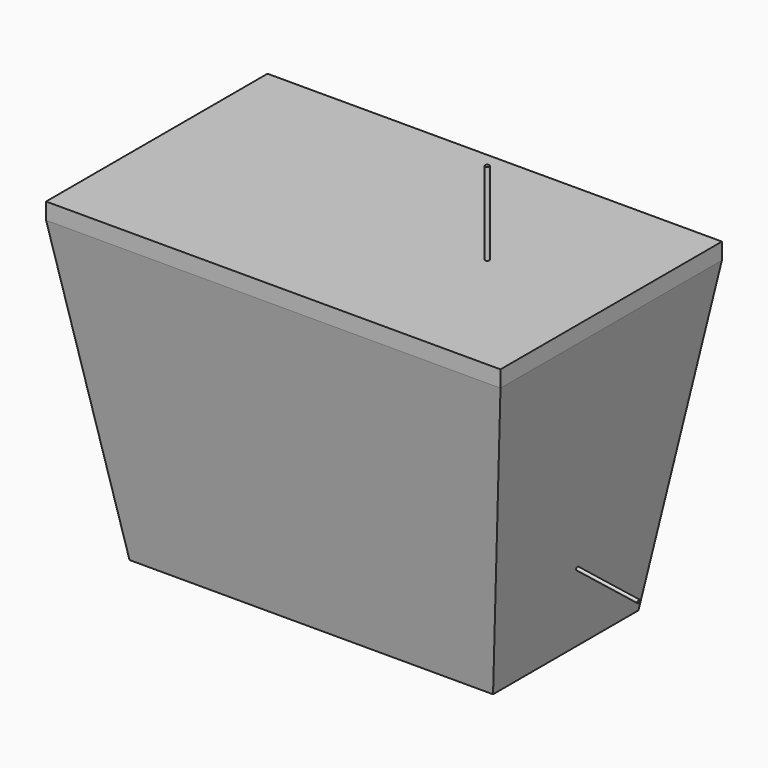
from build123d import *

# Parameters (mm, degrees)
F2_W      = 440
F2_H      = 220
F3_W      = 550
F3_H      = 335
F5_T      = -15
F6_R      = 10
F7_DEPTH  = 160
F8_W      = 10
F8_H      = 0.5
F8_W_2    = 310.5556852937
F8_W_3    = 330.5556852937
F8_H_2    = 7.628889712
F8_W_4    = 350.5556852937
F7_FACE_R = 10
F9_DEPTH  = 1
F8_H_3    = 8
F10_DEPTH = 19.05
F11_W     = 0.5
F11_H     = 137.0105478786
F12_DEPTH = 1
F13_R     = 50
F14_DEPTH = 150
F15_R     = 37.5
F16_DEPTH = 30
F17_R     = 5
F18_R     = 40
F19_DEPTH = 20
F20_R     = 18.75
F21_DEPTH = 25
F25_W     = 550
F25_H     = 335
F26_DEPTH = 20
F27_R     = 1.987683668
F28_DEPTH = 75
F29_R     = 2.5
F30_DEPTH = 100


with BuildPart() as f4:
    # F2 (on offset) → F4 section 0
    with BuildSketch(Plane.XY.offset(-167.5)):
        Rectangle(F2_W, F2_H)
    # F3 (on offset) → F4 section 1
    with BuildSketch(Plane.XY.offset(200)):
        Rectangle(F3_W, F3_H)
    loft()

    # F5
    f5_openings = [f4.faces().sort_by_distance(p)[0] for p in [
        (0, 0, 200),
    ]]
    offset(amount=F5_T, openings=f5_openings)

    # F6 (on face) → F7 (join)
    with BuildSketch(Plane.XY.offset(-152.5)):
        with Locations((-155.2778426469, 48.564444856)):
            Circle(F6_R)
        with Locations((-155.2778426469, -48.564444856)):
            Circle(F6_R)
        with Locations((155.2778426469, 48.564444856)):
            Circle(F6_R)
        with Locations((155.2778426469, -48.564444856)):
            Circle(F6_R)
    extrude(amount=F7_DEPTH)

    # F8 (on face) + F7_face (on face) + F6 (on face) → F9 (join)
    with BuildSketch(Plane.XY.offset(7.5)):
        Polygon((-165.2778426469, -58.564444856), (-165.2778426469, -50.935555144), (-175.2778426469, -50.935555144), (-175.2778426469, -58.935555144), (175.2778426469, -58.935555144), (175.2778426469, -50.935555144), (165.2778426469, -50.935555144), (165.2778426469, -58.564444856), align=None)
        with Locations((-170.2778426469, 0.314444856)):
            Rectangle(F8_W, F8_H)
        with Locations((-170.2778426469, 25.814444856)):
            Rectangle(F8_W, F8_H)
        with Locations((160.2778426469, 25.814444856)):
            Rectangle(F8_W, F8_H)
        with Locations((-160.2778426469, 25.814444856)):
            Rectangle(F8_W, F8_H)
        with Locations((-160.2778426469, -33.685555144)):
            Rectangle(F8_W, F8_H)
        with Locations((-160.2778426469, 0.314444856)):
            Rectangle(F8_W, F8_H)
        with Locations((0, 8.814444856)):
            Rectangle(F8_W_2, F8_H)
        with Locations((0, -25.185555144)):
            Rectangle(F8_W_2, F8_H)
        with Locations((-160.2778426469, 34.314444856)):
            Rectangle(F8_W, F8_H)
        with BuildLine():
            ThreePointArc((-145.7384506327, 51.564444856), (-145.6636664989, 51.3153750614), (-145.5953842813, 51.064444856))
            Line((-145.5953842813, 51.064444856), (165.2778426469, 51.064444856))
            Line((165.2778426469, 51.064444856), (165.2778426469, 51.564444856))
            Line((165.2778426469, 51.564444856), (-145.7384506327, 51.564444856))
        make_face()
        with Locations((160.2778426469, 0.314444856)):
            Rectangle(F8_W, F8_H)
        with Locations((-160.2778426469, -16.685555144)):
            Rectangle(F8_W, F8_H)
        with Locations((160.2778426469, -8.185555144)):
            Rectangle(F8_W, F8_H)
        with Locations((-170.2778426469, -42.185555144)):
            Rectangle(F8_W, F8_H)
        with Locations((160.2778426469, -25.185555144)):
            Rectangle(F8_W, F8_H)
        with Locations((-160.2778426469, -8.185555144)):
            Rectangle(F8_W, F8_H)
        with Locations((0, -42.185555144)):
            Rectangle(F8_W_2, F8_H)
        with Locations((-170.2778426469, 8.814444856)):
            Rectangle(F8_W, F8_H)
        with Locations((0, 0.314444856)):
            Rectangle(F8_W_2, F8_H)
        with Locations((160.2778426469, -16.685555144)):
            Rectangle(F8_W, F8_H)
        with Locations((160.2778426469, 8.814444856)):
            Rectangle(F8_W, F8_H)
        with Locations((0, -33.685555144)):
            Rectangle(F8_W_2, F8_H)
        with Locations((-170.2778426469, -8.185555144)):
            Rectangle(F8_W, F8_H)
        with Locations((-160.2778426469, 17.314444856)):
            Rectangle(F8_W, F8_H)
        with Locations((0, 34.314444856)):
            Rectangle(F8_W_2, F8_H)
        with Locations((-170.2778426469, -16.685555144)):
            Rectangle(F8_W, F8_H)
        with Locations((160.2778426469, -33.685555144)):
            Rectangle(F8_W, F8_H)
        with Locations((160.2778426469, 34.314444856)):
            Rectangle(F8_W, F8_H)
        with BuildLine():
            Line((-145.2778426469, 48.564444856), (-155.2778426469, 48.564444856))
            Line((-155.2778426469, 48.564444856), (-155.2778426469, 43.064444856))
            Line((-155.2778426469, 43.064444856), (-146.9261961026, 43.064444856))
            ThreePointArc((-146.9261961026, 43.064444856), (-145.6987908816, 45.6935970233), (-145.2778426469, 48.564444856))
        make_face()
        with Locations((0, -54.75)):
            Rectangle(F8_W_3, F8_H_2)
        with BuildLine():
            Line((155.2778426469, 43.064444856), (-146.9261961026, 43.064444856))
            ThreePointArc((-146.9261961026, 43.064444856), (-147.0981980227, 42.8117573255), (-147.2778426469, 42.564444856))
            Line((-147.2778426469, 42.564444856), (155.2778426469, 42.564444856))
            Line((155.2778426469, 42.564444856), (155.2778426469, 43.064444856))
        make_face()
        with BuildLine():
            Line((-164.817234661, 51.564444856), (-145.7384506327, 51.564444856))
            ThreePointArc((-145.7384506327, 51.564444856), (-149.3617628638, 56.6267026043), (-155.2778426469, 58.564444856))
            ThreePointArc((-155.2778426469, 58.564444856), (-161.19392243, 56.6267026043), (-164.817234661, 51.564444856))
        make_face()
        with Locations((0, 25.814444856)):
            Rectangle(F8_W_2, F8_H)
        with Locations((0, -8.185555144)):
            Rectangle(F8_W_2, F8_H)
        with Locations((160.2778426469, 42.814444856)):
            Rectangle(F8_W, F8_H)
        with Locations((160.2778426469, 17.314444856)):
            Rectangle(F8_W, F8_H)
        with Locations((-170.2778426469, -50.685555144)):
            Rectangle(F8_W, F8_H)
        with Locations((-170.2778426469, 17.314444856)):
            Rectangle(F8_W, F8_H)
        with Locations((-170.2778426469, 51.314444856)):
            Rectangle(F8_W, F8_H)
        with Locations((-160.2778426469, -25.185555144)):
            Rectangle(F8_W, F8_H)
        with Locations((-160.2778426469, 8.814444856)):
            Rectangle(F8_W, F8_H)
        with Locations((160.2778426469, -42.185555144)):
            Rectangle(F8_W, F8_H)
        with Locations((-170.2778426469, 34.314444856)):
            Rectangle(F8_W, F8_H)
        with Locations((-170.2778426469, -33.685555144)):
            Rectangle(F8_W, F8_H)
        with BuildLine():
            Line((-155.2778426469, 42.564444856), (-155.2778426469, 43.064444856))
            Line((-155.2778426469, 43.064444856), (-163.6294891911, 43.064444856))
            ThreePointArc((-163.6294891911, 43.064444856), (-163.457487271, 42.8117573255), (-163.2778426469, 42.564444856))
            Line((-163.2778426469, 42.564444856), (-155.2778426469, 42.564444856))
        make_face()
        with Locations((-170.2778426469, -25.185555144)):
            Rectangle(F8_W, F8_H)
        with Locations((-170.2778426469, 42.814444856)):
            Rectangle(F8_W, F8_H)
        with Locations((0, -16.685555144)):
            Rectangle(F8_W_2, F8_H)
        with Locations((0, 17.314444856)):
            Rectangle(F8_W_2, F8_H)
        with BuildLine():
            Line((-147.2778426469, 42.564444856), (-155.2778426469, 42.564444856))
            Line((-155.2778426469, 42.564444856), (-155.2778426469, 38.564444856))
            ThreePointArc((-155.2778426469, 38.564444856), (-150.8057066919, 39.620172946), (-147.2778426469, 42.564444856))
        make_face()
        with Locations((-160.2778426469, -42.185555144)):
            Rectangle(F8_W, F8_H)
        with BuildLine():
            Line((-155.2778426469, 43.064444856), (-155.2778426469, 48.564444856))
            Line((-155.2778426469, 48.564444856), (-145.2778426469, 48.564444856))
            ThreePointArc((-145.2778426469, 48.564444856), (-145.3575456842, 49.8244877808), (-145.5953842813, 51.064444856))
            Line((-145.5953842813, 51.064444856), (-164.9603010124, 51.064444856))
            ThreePointArc((-164.9603010124, 51.064444856), (-165.1981396095, 49.8244877808), (-165.2778426469, 48.564444856))
            ThreePointArc((-165.2778426469, 48.564444856), (-164.8568944121, 45.6935970233), (-163.6294891911, 43.064444856))
            Line((-163.6294891911, 43.064444856), (-155.2778426469, 43.064444856))
        make_face()
        with BuildLine():
            Line((-146.9261961026, 43.064444856), (-155.2778426469, 43.064444856))
            Line((-155.2778426469, 43.064444856), (-155.2778426469, 42.564444856))
            Line((-155.2778426469, 42.564444856), (-147.2778426469, 42.564444856))
            ThreePointArc((-147.2778426469, 42.564444856), (-147.0981980227, 42.8117573255), (-146.9261961026, 43.064444856))
        make_face()
        with Locations((0, -50.685555144)):
            Rectangle(F8_W_3, F8_H)
        with BuildLine():
            Line((-155.2778426469, 38.564444856), (-155.2778426469, 42.564444856))
            Line((-155.2778426469, 42.564444856), (-163.2778426469, 42.564444856))
            ThreePointArc((-163.2778426469, 42.564444856), (-159.7499786019, 39.620172946), (-155.2778426469, 38.564444856))
        make_face()
        with BuildLine():
            Line((-164.9603010124, 51.064444856), (-145.5953842813, 51.064444856))
            ThreePointArc((-145.5953842813, 51.064444856), (-145.6636664989, 51.3153750614), (-145.7384506327, 51.564444856))
            Line((-145.7384506327, 51.564444856), (-164.817234661, 51.564444856))
            ThreePointArc((-164.817234661, 51.564444856), (-164.8920187949, 51.3153750614), (-164.9603010124, 51.064444856))
        make_face()
        with BuildLine():
            ThreePointArc((-163.2778426469, 42.564444856), (-163.457487271, 42.8117573255), (-163.6294891911, 43.064444856))
            Line((-163.6294891911, 43.064444856), (-165.2778426469, 43.064444856))
            Line((-165.2778426469, 43.064444856), (-165.2778426469, 42.564444856))
            Line((-165.2778426469, 42.564444856), (-163.2778426469, 42.564444856))
        make_face()
        with BuildLine():
            Line((-165.2778426469, 51.064444856), (-164.9603010124, 51.064444856))
            ThreePointArc((-164.9603010124, 51.064444856), (-164.8920187949, 51.3153750614), (-164.817234661, 51.564444856))
            Line((-164.817234661, 51.564444856), (-165.2778426469, 51.564444856))
            Line((-165.2778426469, 51.564444856), (-165.2778426469, 51.064444856))
        make_face()
        with Locations((0, 68.314444856)):
            Rectangle(F8_W_4, F8_H)
        with Locations((0, 59.814444856)):
            Rectangle(F8_W_4, F8_H)
    with BuildSketch(Plane(origin=(-155.2778426469, 48.564444856, 7.5), x_dir=(1, 0, 0), z_dir=(0, 0, 1))):
        with Locations((310.5556852937, -97.128889712)):
            Circle(F7_FACE_R)
        with Locations((0, -97.128889712)):
            Circle(F7_FACE_R)
        Circle(F7_FACE_R)
        with Locations((310.5556852937, 0)):
            Circle(F7_FACE_R)
    with BuildSketch(Plane.XY.offset(-152.5)):
        with Locations((-155.2778426469, -48.564444856)):
            Circle(F6_R)
        with Locations((155.2778426469, -48.564444856)):
            Circle(F6_R)
        with Locations((155.2778426469, 48.564444856)):
            Circle(F6_R)
        with Locations((-155.2778426469, 48.564444856)):
            Circle(F6_R)
    extrude(amount=-F9_DEPTH)

    # F18 (on face) → F19 (join)
    with BuildSketch(Plane.XY.offset(-152.5)):
        Circle(F18_R)
    extrude(amount=F19_DEPTH)

    # F20 (on face) → F21 (join)
    with BuildSketch(Plane.XY.offset(-132.5)):
        Circle(F20_R)
    extrude(amount=F21_DEPTH)

    # F23 (on face) → F24 (revolve)
    with BuildSketch(Plane(origin=(0, 0, 0), x_dir=(0, -1, 0), z_dir=(-1, 0, 0))):
        with BuildLine():
            Line((0, -40), (0, -120))
            ThreePointArc((0, -120), (45.3792520632, -80), (0, -40))
        make_face()
    revolve(axis=Axis((0, 0, -80), (0, 0, -1)))

    # F25 (on face) → F26 (join)
    with BuildSketch(Plane.XY.offset(200)):
        Rectangle(F25_W, F25_H)
    extrude(amount=F26_DEPTH)

    # F27 (on face) → F28 (join, symmetric)
    with BuildSketch(Plane(origin=(239.6992259992, 0, -35.8733535509), x_dir=(0, 1, 0), z_dir=(0.9889856463, 0, -0.1480114573))):
        with Locations((0, -38.0925751513)):
            Circle(F27_R)
    extrude(amount=F28_DEPTH, both=True)


with BuildPart() as f10:
    # F8 (on face) → F10 (new body)
    with BuildSketch(Plane.XY.offset(7.5)):
        with Locations((0, -64.564444856)):
            Rectangle(F8_W_4, F8_H_3)
    extrude(amount=-F10_DEPTH)


with BuildPart() as f10b:
    # F8 (on face) → F10, piece 2 (new body)
    with BuildSketch(Plane.XY.offset(7.5)):
        Polygon((-165.2778426469, -58.564444856), (-165.2778426469, -50.935555144), (-175.2778426469, -50.935555144), (-175.2778426469, -58.935555144), (175.2778426469, -58.935555144), (175.2778426469, -50.935555144), (165.2778426469, -50.935555144), (165.2778426469, -58.564444856), align=None)
    extrude(amount=-F10_DEPTH)


with BuildPart() as f10c:
    # F8 (on face) → F10, piece 3 (new body)
    with BuildSketch(Plane.XY.offset(7.5)):
        with Locations((170.2778426469, -46.435555144)):
            Rectangle(F8_W, F8_H_3)
    extrude(amount=-F10_DEPTH)


with BuildPart() as f10d:
    # F8 (on face) → F10, piece 4 (new body)
    with BuildSketch(Plane.XY.offset(7.5)):
        with Locations((170.2778426469, -37.935555144)):
            Rectangle(F8_W, F8_H_3)
    extrude(amount=-F10_DEPTH)


with BuildPart() as f10e:
    # F8 (on face) → F10, piece 5 (new body)
    with BuildSketch(Plane.XY.offset(7.5)):
        with Locations((170.2778426469, -29.435555144)):
            Rectangle(F8_W, F8_H_3)
    extrude(amount=-F10_DEPTH)


with BuildPart() as f10f:
    # F8 (on face) → F10, piece 6 (new body)
    with BuildSketch(Plane.XY.offset(7.5)):
        with Locations((170.2778426469, -20.935555144)):
            Rectangle(F8_W, F8_H_3)
    extrude(amount=-F10_DEPTH)


with BuildPart() as f10g:
    # F8 (on face) → F10, piece 7 (new body)
    with BuildSketch(Plane.XY.offset(7.5)):
        with Locations((170.2778426469, -12.435555144)):
            Rectangle(F8_W, F8_H_3)
    extrude(amount=-F10_DEPTH)


with BuildPart() as f10h:
    # F8 (on face) → F10, piece 8 (new body)
    with BuildSketch(Plane.XY.offset(7.5)):
        with Locations((170.2778426469, -3.935555144)):
            Rectangle(F8_W, F8_H_3)
    extrude(amount=-F10_DEPTH)


with BuildPart() as f10i:
    # F8 (on face) → F10, piece 9 (new body)
    with BuildSketch(Plane.XY.offset(7.5)):
        with Locations((170.2778426469, 4.564444856)):
            Rectangle(F8_W, F8_H_3)
    extrude(amount=-F10_DEPTH)


with BuildPart() as f10j:
    # F8 (on face) → F10, piece 10 (new body)
    with BuildSketch(Plane.XY.offset(7.5)):
        with Locations((170.2778426469, 13.064444856)):
            Rectangle(F8_W, F8_H_3)
    extrude(amount=-F10_DEPTH)


with BuildPart() as f10k:
    # F8 (on face) → F10, piece 11 (new body)
    with BuildSketch(Plane.XY.offset(7.5)):
        with Locations((170.2778426469, 21.564444856)):
            Rectangle(F8_W, F8_H_3)
    extrude(amount=-F10_DEPTH)


with BuildPart() as f10l:
    # F8 (on face) → F10, piece 12 (new body)
    with BuildSketch(Plane.XY.offset(7.5)):
        with Locations((170.2778426469, 30.064444856)):
            Rectangle(F8_W, F8_H_3)
    extrude(amount=-F10_DEPTH)


with BuildPart() as f10m:
    # F8 (on face) → F10, piece 13 (new body)
    with BuildSketch(Plane.XY.offset(7.5)):
        with Locations((170.2778426469, 38.564444856)):
            Rectangle(F8_W, F8_H_3)
    extrude(amount=-F10_DEPTH)


with BuildPart() as f10n:
    # F8 (on face) → F10, piece 14 (new body)
    with BuildSketch(Plane.XY.offset(7.5)):
        with Locations((170.2778426469, 47.064444856)):
            Rectangle(F8_W, F8_H_3)
    extrude(amount=-F10_DEPTH)


with BuildPart() as f10o:
    # F8 (on face) → F10, piece 15 (new body)
    with BuildSketch(Plane.XY.offset(7.5)):
        Polygon((165.2778426469, 58.564444856), (165.2778426469, 51.564444856), (175.2778426469, 51.564444856), (175.2778426469, 59.564444856), (-175.2778426469, 59.564444856), (-175.2778426469, 51.564444856), (-165.2778426469, 51.564444856), (-165.2778426469, 58.564444856), (-155.2778426469, 58.564444856), align=None)
    extrude(amount=-F10_DEPTH)


with BuildPart() as f10p:
    # F8 (on face) → F10, piece 16 (new body)
    with BuildSketch(Plane.XY.offset(7.5)):
        with Locations((0, 64.064444856)):
            Rectangle(F8_W_4, F8_H_3)
    extrude(amount=-F10_DEPTH)


with BuildPart() as f10q:
    # F8 (on face) → F10, piece 17 (new body)
    with BuildSketch(Plane.XY.offset(7.5)):
        Polygon((-175.2778426469, 43.064444856), (-165.2778426469, 43.064444856), (-165.2778426469, 48.564444856), (-165.2778426469, 51.064444856), (-175.2778426469, 51.064444856), align=None)
    extrude(amount=-F10_DEPTH)


with BuildPart() as f10r:
    # F8 (on face) → F10, piece 18 (new body)
    with BuildSketch(Plane.XY.offset(7.5)):
        with Locations((-170.2778426469, 38.564444856)):
            Rectangle(F8_W, F8_H_3)
    extrude(amount=-F10_DEPTH)


with BuildPart() as f10s:
    # F8 (on face) → F10, piece 19 (new body)
    with BuildSketch(Plane.XY.offset(7.5)):
        with Locations((-170.2778426469, 30.064444856)):
            Rectangle(F8_W, F8_H_3)
    extrude(amount=-F10_DEPTH)


with BuildPart() as f10t:
    # F8 (on face) → F10, piece 20 (new body)
    with BuildSketch(Plane.XY.offset(7.5)):
        with Locations((-170.2778426469, 21.564444856)):
            Rectangle(F8_W, F8_H_3)
    extrude(amount=-F10_DEPTH)


with BuildPart() as f10u:
    # F8 (on face) → F10, piece 21 (new body)
    with BuildSketch(Plane.XY.offset(7.5)):
        with Locations((-170.2778426469, 13.064444856)):
            Rectangle(F8_W, F8_H_3)
    extrude(amount=-F10_DEPTH)


with BuildPart() as f10v:
    # F8 (on face) → F10, piece 22 (new body)
    with BuildSketch(Plane.XY.offset(7.5)):
        with Locations((-170.2778426469, 4.564444856)):
            Rectangle(F8_W, F8_H_3)
    extrude(amount=-F10_DEPTH)


with BuildPart() as f10w:
    # F8 (on face) → F10, piece 23 (new body)
    with BuildSketch(Plane.XY.offset(7.5)):
        with Locations((-170.2778426469, -3.935555144)):
            Rectangle(F8_W, F8_H_3)
    extrude(amount=-F10_DEPTH)


with BuildPart() as f10x:
    # F8 (on face) → F10, piece 24 (new body)
    with BuildSketch(Plane.XY.offset(7.5)):
        with Locations((-170.2778426469, -12.435555144)):
            Rectangle(F8_W, F8_H_3)
    extrude(amount=-F10_DEPTH)


with BuildPart() as f10y:
    # F8 (on face) → F10, piece 25 (new body)
    with BuildSketch(Plane.XY.offset(7.5)):
        with Locations((-170.2778426469, -20.935555144)):
            Rectangle(F8_W, F8_H_3)
    extrude(amount=-F10_DEPTH)


with BuildPart() as f10z:
    # F8 (on face) → F10, piece 26 (new body)
    with BuildSketch(Plane.XY.offset(7.5)):
        with Locations((-170.2778426469, -29.435555144)):
            Rectangle(F8_W, F8_H_3)
    extrude(amount=-F10_DEPTH)


with BuildPart() as f10ba:
    # F8 (on face) → F10, piece 27 (new body)
    with BuildSketch(Plane.XY.offset(7.5)):
        with Locations((-170.2778426469, -37.935555144)):
            Rectangle(F8_W, F8_H_3)
    extrude(amount=-F10_DEPTH)


with BuildPart() as f10bb:
    # F8 (on face) → F10, piece 28 (new body)
    with BuildSketch(Plane.XY.offset(7.5)):
        with Locations((-170.2778426469, -46.435555144)):
            Rectangle(F8_W, F8_H_3)
    extrude(amount=-F10_DEPTH)


with BuildPart() as f12:
    # F11 (on face) → F12 (new body)
    with BuildSketch(Plane.XY.offset(7.5)):
        with Locations((-175.0278426469, -0.4408290833)):
            Rectangle(F11_W, F11_H)
    extrude(amount=-F12_DEPTH)


with BuildPart() as f12b:
    # F11 (on face) → F12, piece 2 (new body)
    with BuildSketch(Plane.XY.offset(7.5)):
        with Locations((-167.0278426469, -0.4408290833)):
            Rectangle(F11_W, F11_H)
    extrude(amount=-F12_DEPTH)


with BuildPart() as f12c:
    # F11 (on face) → F12, piece 3 (new body)
    with BuildSketch(Plane.XY.offset(7.5)):
        with Locations((-159.0278426469, -0.4408290833)):
            Rectangle(F11_W, F11_H)
    extrude(amount=-F12_DEPTH)


with BuildPart() as f12d:
    # F11 (on face) → F12, piece 4 (new body)
    with BuildSketch(Plane.XY.offset(7.5)):
        with Locations((-151.0278426469, -0.4408290833)):
            Rectangle(F11_W, F11_H)
    extrude(amount=-F12_DEPTH)


with BuildPart() as f12e:
    # F11 (on face) → F12, piece 5 (new body)
    with BuildSketch(Plane.XY.offset(7.5)):
        with Locations((-143.0278426469, -0.4408290833)):
            Rectangle(F11_W, F11_H)
    extrude(amount=-F12_DEPTH)


with BuildPart() as f12f:
    # F11 (on face) → F12, piece 6 (new body)
    with BuildSketch(Plane.XY.offset(7.5)):
        with Locations((-135.0278426469, -0.4408290833)):
            Rectangle(F11_W, F11_H)
    extrude(amount=-F12_DEPTH)


with BuildPart() as f12g:
    # F11 (on face) → F12, piece 7 (new body)
    with BuildSketch(Plane.XY.offset(7.5)):
        with Locations((-127.0278426469, -0.4408290833)):
            Rectangle(F11_W, F11_H)
    extrude(amount=-F12_DEPTH)


with BuildPart() as f12h:
    # F11 (on face) → F12, piece 8 (new body)
    with BuildSketch(Plane.XY.offset(7.5)):
        with Locations((-119.0278426469, -0.4408290833)):
            Rectangle(F11_W, F11_H)
    extrude(amount=-F12_DEPTH)


with BuildPart() as f12i:
    # F11 (on face) → F12, piece 9 (new body)
    with BuildSketch(Plane.XY.offset(7.5)):
        with Locations((-111.0278426469, -0.4408290833)):
            Rectangle(F11_W, F11_H)
    extrude(amount=-F12_DEPTH)


with BuildPart() as f12j:
    # F11 (on face) → F12, piece 10 (new body)
    with BuildSketch(Plane.XY.offset(7.5)):
        with Locations((-103.0278426469, -0.4408290833)):
            Rectangle(F11_W, F11_H)
    extrude(amount=-F12_DEPTH)


with BuildPart() as f12k:
    # F11 (on face) → F12, piece 11 (new body)
    with BuildSketch(Plane.XY.offset(7.5)):
        with Locations((-95.0278426469, -0.4408290833)):
            Rectangle(F11_W, F11_H)
    extrude(amount=-F12_DEPTH)


with BuildPart() as f12l:
    # F11 (on face) → F12, piece 12 (new body)
    with BuildSketch(Plane.XY.offset(7.5)):
        with Locations((-87.0278426469, -0.4408290833)):
            Rectangle(F11_W, F11_H)
    extrude(amount=-F12_DEPTH)


with BuildPart() as f12m:
    # F11 (on face) → F12, piece 13 (new body)
    with BuildSketch(Plane.XY.offset(7.5)):
        with Locations((-79.0278426469, -0.4408290833)):
            Rectangle(F11_W, F11_H)
    extrude(amount=-F12_DEPTH)


with BuildPart() as f12n:
    # F11 (on face) → F12, piece 14 (new body)
    with BuildSketch(Plane.XY.offset(7.5)):
        with Locations((-71.0278426469, -0.4408290833)):
            Rectangle(F11_W, F11_H)
    extrude(amount=-F12_DEPTH)


with BuildPart() as f12o:
    # F11 (on face) → F12, piece 15 (new body)
    with BuildSketch(Plane.XY.offset(7.5)):
        with Locations((-63.0278426469, -0.4408290833)):
            Rectangle(F11_W, F11_H)
    extrude(amount=-F12_DEPTH)


with BuildPart() as f12p:
    # F11 (on face) → F12, piece 16 (new body)
    with BuildSketch(Plane.XY.offset(7.5)):
        with Locations((-55.0278426469, -0.4408290833)):
            Rectangle(F11_W, F11_H)
    extrude(amount=-F12_DEPTH)


with BuildPart() as f12q:
    # F11 (on face) → F12, piece 17 (new body)
    with BuildSketch(Plane.XY.offset(7.5)):
        with Locations((-47.0278426469, -0.4408290833)):
            Rectangle(F11_W, F11_H)
    extrude(amount=-F12_DEPTH)


with BuildPart() as f12r:
    # F11 (on face) → F12, piece 18 (new body)
    with BuildSketch(Plane.XY.offset(7.5)):
        with Locations((-39.0278426469, -0.4408290833)):
            Rectangle(F11_W, F11_H)
    extrude(amount=-F12_DEPTH)


with BuildPart() as f12s:
    # F11 (on face) → F12, piece 19 (new body)
    with BuildSketch(Plane.XY.offset(7.5)):
        with Locations((-31.0278426469, -0.4408290833)):
            Rectangle(F11_W, F11_H)
    extrude(amount=-F12_DEPTH)


with BuildPart() as f12t:
    # F11 (on face) → F12, piece 20 (new body)
    with BuildSketch(Plane.XY.offset(7.5)):
        with Locations((-23.0278426469, -0.4408290833)):
            Rectangle(F11_W, F11_H)
    extrude(amount=-F12_DEPTH)


with BuildPart() as f12u:
    # F11 (on face) → F12, piece 21 (new body)
    with BuildSketch(Plane.XY.offset(7.5)):
        with Locations((-15.0278426469, -0.4408290833)):
            Rectangle(F11_W, F11_H)
    extrude(amount=-F12_DEPTH)


with BuildPart() as f12v:
    # F11 (on face) → F12, piece 22 (new body)
    with BuildSketch(Plane.XY.offset(7.5)):
        with Locations((-7.0278426469, -0.4408290833)):
            Rectangle(F11_W, F11_H)
    extrude(amount=-F12_DEPTH)


with BuildPart() as f12w:
    # F11 (on face) → F12, piece 23 (new body)
    with BuildSketch(Plane.XY.offset(7.5)):
        with Locations((0.9721573531, -0.4408290833)):
            Rectangle(F11_W, F11_H)
    extrude(amount=-F12_DEPTH)


with BuildPart() as f12x:
    # F11 (on face) → F12, piece 24 (new body)
    with BuildSketch(Plane.XY.offset(7.5)):
        with Locations((8.9721573531, -0.4408290833)):
            Rectangle(F11_W, F11_H)
    extrude(amount=-F12_DEPTH)


with BuildPart() as f12y:
    # F11 (on face) → F12, piece 25 (new body)
    with BuildSketch(Plane.XY.offset(7.5)):
        with Locations((16.9721573531, -0.4408290833)):
            Rectangle(F11_W, F11_H)
    extrude(amount=-F12_DEPTH)


with BuildPart() as f12z:
    # F11 (on face) → F12, piece 26 (new body)
    with BuildSketch(Plane.XY.offset(7.5)):
        with Locations((24.9721573531, -0.4408290833)):
            Rectangle(F11_W, F11_H)
    extrude(amount=-F12_DEPTH)


with BuildPart() as f12ba:
    # F11 (on face) → F12, piece 27 (new body)
    with BuildSketch(Plane.XY.offset(7.5)):
        with Locations((32.9721573531, -0.4408290833)):
            Rectangle(F11_W, F11_H)
    extrude(amount=-F12_DEPTH)


with BuildPart() as f12bb:
    # F11 (on face) → F12, piece 28 (new body)
    with BuildSketch(Plane.XY.offset(7.5)):
        with Locations((40.9721573531, -0.4408290833)):
            Rectangle(F11_W, F11_H)
    extrude(amount=-F12_DEPTH)


with BuildPart() as f12bc:
    # F11 (on face) → F12, piece 29 (new body)
    with BuildSketch(Plane.XY.offset(7.5)):
        with Locations((48.9721573531, -0.4408290833)):
            Rectangle(F11_W, F11_H)
    extrude(amount=-F12_DEPTH)


with BuildPart() as f12bd:
    # F11 (on face) → F12, piece 30 (new body)
    with BuildSketch(Plane.XY.offset(7.5)):
        with Locations((56.9721573531, -0.4408290833)):
            Rectangle(F11_W, F11_H)
    extrude(amount=-F12_DEPTH)


with BuildPart() as f12be:
    # F11 (on face) → F12, piece 31 (new body)
    with BuildSketch(Plane.XY.offset(7.5)):
        with Locations((64.9721573531, -0.4408290833)):
            Rectangle(F11_W, F11_H)
    extrude(amount=-F12_DEPTH)


with BuildPart() as f12bf:
    # F11 (on face) → F12, piece 32 (new body)
    with BuildSketch(Plane.XY.offset(7.5)):
        with Locations((72.9721573531, -0.4408290833)):
            Rectangle(F11_W, F11_H)
    extrude(amount=-F12_DEPTH)


with BuildPart() as f12bg:
    # F11 (on face) → F12, piece 33 (new body)
    with BuildSketch(Plane.XY.offset(7.5)):
        with Locations((80.9721573531, -0.4408290833)):
            Rectangle(F11_W, F11_H)
    extrude(amount=-F12_DEPTH)


with BuildPart() as f12bh:
    # F11 (on face) → F12, piece 34 (new body)
    with BuildSketch(Plane.XY.offset(7.5)):
        with Locations((88.9721573531, -0.4408290833)):
            Rectangle(F11_W, F11_H)
    extrude(amount=-F12_DEPTH)


with BuildPart() as f12bi:
    # F11 (on face) → F12, piece 35 (new body)
    with BuildSketch(Plane.XY.offset(7.5)):
        with Locations((96.9721573531, -0.4408290833)):
            Rectangle(F11_W, F11_H)
    extrude(amount=-F12_DEPTH)


with BuildPart() as f12bj:
    # F11 (on face) → F12, piece 36 (new body)
    with BuildSketch(Plane.XY.offset(7.5)):
        with Locations((104.9721573531, -0.4408290833)):
            Rectangle(F11_W, F11_H)
    extrude(amount=-F12_DEPTH)


with BuildPart() as f12bk:
    # F11 (on face) → F12, piece 37 (new body)
    with BuildSketch(Plane.XY.offset(7.5)):
        with Locations((112.9721573531, -0.4408290833)):
            Rectangle(F11_W, F11_H)
    extrude(amount=-F12_DEPTH)


with BuildPart() as f12bl:
    # F11 (on face) → F12, piece 38 (new body)
    with BuildSketch(Plane.XY.offset(7.5)):
        with Locations((120.9721573531, -0.4408290833)):
            Rectangle(F11_W, F11_H)
    extrude(amount=-F12_DEPTH)


with BuildPart() as f12bm:
    # F11 (on face) → F12, piece 39 (new body)
    with BuildSketch(Plane.XY.offset(7.5)):
        with Locations((128.9721573531, -0.4408290833)):
            Rectangle(F11_W, F11_H)
    extrude(amount=-F12_DEPTH)


with BuildPart() as f12bn:
    # F11 (on face) → F12, piece 40 (new body)
    with BuildSketch(Plane.XY.offset(7.5)):
        with Locations((136.9721573531, -0.4408290833)):
            Rectangle(F11_W, F11_H)
    extrude(amount=-F12_DEPTH)


with BuildPart() as f12bo:
    # F11 (on face) → F12, piece 41 (new body)
    with BuildSketch(Plane.XY.offset(7.5)):
        with Locations((144.9721573531, -0.4408290833)):
            Rectangle(F11_W, F11_H)
    extrude(amount=-F12_DEPTH)


with BuildPart() as f12bp:
    # F11 (on face) → F12, piece 42 (new body)
    with BuildSketch(Plane.XY.offset(7.5)):
        with Locations((152.9721573531, -0.4408290833)):
            Rectangle(F11_W, F11_H)
    extrude(amount=-F12_DEPTH)


with BuildPart() as f12bq:
    # F11 (on face) → F12, piece 43 (new body)
    with BuildSketch(Plane.XY.offset(7.5)):
        with Locations((160.9721573531, -0.4408290833)):
            Rectangle(F11_W, F11_H)
    extrude(amount=-F12_DEPTH)


with BuildPart() as f12br:
    # F11 (on face) → F12, piece 44 (new body)
    with BuildSketch(Plane.XY.offset(7.5)):
        with Locations((168.9721573531, -0.4408290833)):
            Rectangle(F11_W, F11_H)
    extrude(amount=-F12_DEPTH)


with BuildPart() as f14:
    # F13 (on face) → F14 (new body)
    with BuildSketch(Plane.XY.offset(7.5)):
        Circle(F13_R)
    extrude(amount=F14_DEPTH)

    # F15 (on face) → F16 (join)
    with BuildSketch(Plane.XY.offset(157.5)):
        Circle(F15_R)
    extrude(amount=F16_DEPTH)

    # F17
    f17_edges = [f14.edges().sort_by_distance(p)[0] for p in [
        (-50, 0, 157.5),
        (-37.5, 0, 157.5),
        (-50, 0, 7.5),
        (-37.5, 0, 187.5),
    ]]
    fillet(f17_edges, radius=F17_R)


with BuildPart() as f30:
    # F29 (on face) → F30 (new body, symmetric)
    with BuildSketch(Plane.XY.offset(220)):
        with Locations((125, 0)):
            Circle(F29_R)
    extrude(amount=F30_DEPTH, both=True)


solid = Compound([f4.part, f10.part, f10b.part, f10c.part, f10d.part, f10e.part, f10f.part, f10g.part, f10h.part, f10i.part, f10j.part, f10k.part, f10l.part, f10m.part, f10n.part, f10o.part, f10p.part, f10q.part, f10r.part, f10s.part, f10t.part, f10u.part, f10v.part, f10w.part, f10x.part, f10y.part, f10z.part, f10ba.part, f10bb.part, f12.part, f12b.part, f12c.part, f12d.part, f12e.part, f12f.part, f12g.part, f12h.part, f12i.part, f12j.part, f12k.part, f12l.part, f12m.part, f12n.part, f12o.part, f12p.part, f12q.part, f12r.part, f12s.part, f12t.part, f12u.part, f12v.part, f12w.part, f12x.part, f12y.part, f12z.part, f12ba.part, f12bb.part, f12bc.part, f12bd.part, f12be.part, f12bf.part, f12bg.part, f12bh.part, f12bi.part, f12bj.part, f12bk.part, f12bl.part, f12bm.part, f12bn.part, f12bo.part, f12bp.part, f12bq.part, f12br.part, f14.part, f30.part])
